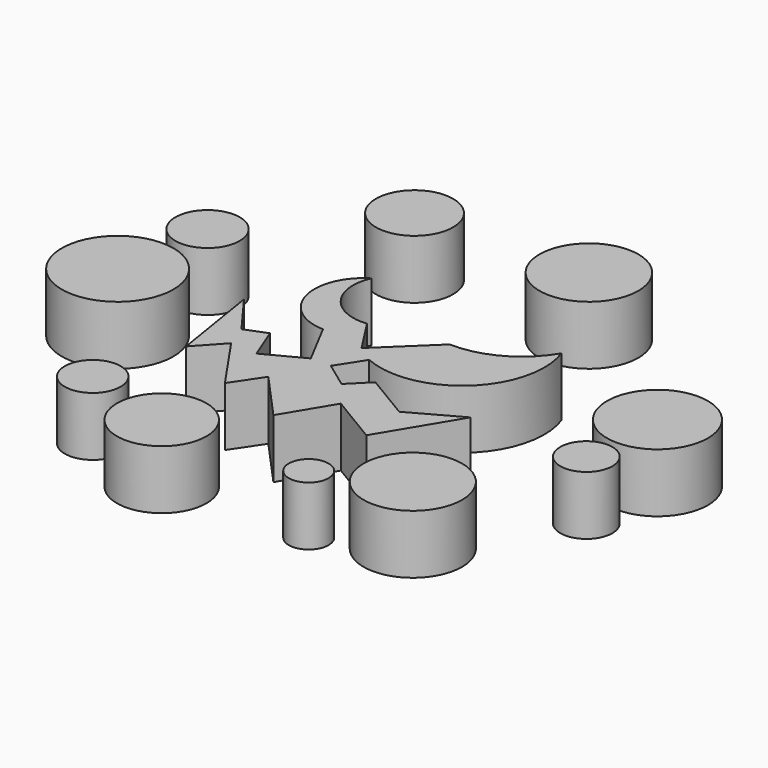
from build123d import *

# Parameters (mm, degrees)
F1_DEPTH = 3.175
F0_R     = 3.0058400938
F0_R_2   = 1.7297628863
F0_R_3   = 2.0789147202
F0_R_4   = 2.6623124831
F0_R_5   = 2.7142518638
F0_R_6   = 1.4028991856
F0_R_7   = 2.6523027823
F0_R_8   = 1.0713376485
F0_R_9   = 2.4079005593
F0_R_10  = 1.503555761


# Not quite as in the source:
# - a feature names something its author has since deleted; it is built from what else it names


with BuildPart() as f1:
    # F0 (on Top) → F1 (new body)
    with BuildSketch(Plane.XY):
        with BuildLine():
            Line((-6.1197558618, -0.8369509036), (-7.7342026882, 1.354082565))
            Line((-7.7342026882, 1.354082565), (-6.9561327472, -3.5171294496))
            Line((-6.9561327472, -3.5171294496), (-5.6584882394, -2.105442362))
            Line((-5.6584882394, -2.105442362), (-3.5983910284, -5.0996665728))
            Line((-3.5983910284, -5.0996665728), (-2.5265401718, -3.5171294496))
            Line((-2.5265401718, -3.5171294496), (-0.1793996592, -6.1098384625))
            Line((-0.1793996592, -6.1098384625), (1.3758814801, -3.5171294496))
            Line((1.3758814801, -3.5171294496), (4.0140271882, -5.0996665728))
            Line((4.0140271882, -5.0996665728), (6.4169475934, -1.0939127355))
            Line((6.4169475934, -1.0939127355), (3.7565478899, -2.5639539262))
            Line((3.7565478899, -2.5639539262), (1.296967469, -1.0939127355))
            Line((1.296967469, -1.0939127355), (0.2841313167, -2.105442362))
            Line((0.2841313167, -2.105442362), (-1.1021959199, -1.0939127355))
            Line((-1.1021959199, -1.0939127355), (-0.1793996592, 0.3343850841))
            ThreePointArc((-0.1793996592, 0.3343850841), (4.5929798172, 1.1518206005), (5.7579467259, 5.8514651393))
            ThreePointArc((5.7579467259, 5.8514651393), (3.9849443716, 4.1276898045), (1.5817080986, 3.5451143423))
            Line((1.5817080986, 3.5451143423), (-1.1021959199, 0.9732797643))
            Line((-1.1021959199, 0.9732797643), (-2.3142797951, 2.8532103717))
            ThreePointArc((-2.3142797951, 2.8532103717), (-4.499498148, 3.8197245452), (-4.735944538, 6.1974171246))
            ThreePointArc((-4.735944538, 6.1974171246), (-5.9170454131, 3.2620282391), (-3.4369527023, 1.2971752339))
            Line((-3.4369527023, 1.2971752339), (-2.1779222215, -1.0939127355))
            Line((-2.1779222215, -1.0939127355), (-4.2390126121, -2.1791825618))
            Line((-4.2390126121, -2.1791825618), (-4.9504833449, -0.3756800361))
            Line((-4.9504833449, -0.3756800361), (-6.1197558618, -0.8369509036))
        make_face()
    extrude(amount=F1_DEPTH)


with BuildPart() as f1b:
    # F0 (on Top) → F1, piece 2 (new body)
    with BuildSketch(Plane.XY):
        with Locations((-13.6153940494, 0.2009075893)):
            Circle(F0_R)
    extrude(amount=F1_DEPTH)


with BuildPart() as f1c:
    # F0 (on Top) → F1, piece 3 (new body)
    with BuildSketch(Plane.XY):
        with Locations((-12.9234905016, 5.3901949799)):
            Circle(F0_R_2)
    extrude(amount=F1_DEPTH)


with BuildPart() as f1d:
    # F0 (on Top) → F1, piece 4 (new body)
    with BuildSketch(Plane.XY):
        with Locations((-7.0422970263, 11.9632928487)):
            Circle(F0_R_3)
    extrude(amount=F1_DEPTH)


with BuildPart() as f1e:
    # F0 (on Top) → F1, piece 5 (new body)
    with BuildSketch(Plane.XY):
        with Locations((2.0677854507, 12.3092456796)):
            Circle(F0_R_4)
    extrude(amount=F1_DEPTH)


with BuildPart() as f1f:
    # F0 (on Top) → F1, piece 6 (new body)
    with BuildSketch(Plane.XY):
        with Locations((12.6769982713, 3.6604325164)):
            Circle(F0_R_5)
    extrude(amount=F1_DEPTH)


with BuildPart() as f1g:
    # F0 (on Top) → F1, piece 7 (new body)
    with BuildSketch(Plane.XY):
        with Locations((12.4463619232, -0.8369509036)):
            Circle(F0_R_6)
    extrude(amount=F1_DEPTH)


with BuildPart() as f1h:
    # F0 (on Top) → F1, piece 8 (new body)
    with BuildSketch(Plane.XY):
        with Locations((8.1796131601, -7.1794132698)):
            Circle(F0_R_7)
    extrude(amount=F1_DEPTH)


with BuildPart() as f1i:
    # F0 (on Top) → F1, piece 9 (new body)
    with BuildSketch(Plane.XY):
        with Locations((4.1434990539, -9.1398103902)):
            Circle(F0_R_8)
    extrude(amount=F1_DEPTH)


with BuildPart() as f1j:
    # F0 (on Top) → F1, piece 10 (new body)
    with BuildSketch(Plane.XY):
        with Locations((-3.5827695623, -9.3704450471)):
            Circle(F0_R_9)
    extrude(amount=F1_DEPTH)


with BuildPart() as f1k:
    # F0 (on Top) → F1, piece 11 (new body)
    with BuildSketch(Plane.XY):
        with Locations((-8.3107901761, -8.1019535886)):
            Circle(F0_R_10)
    extrude(amount=F1_DEPTH)


solid = Compound([f1.part, f1b.part, f1c.part, f1d.part, f1e.part, f1f.part, f1g.part, f1h.part, f1i.part, f1j.part, f1k.part])
